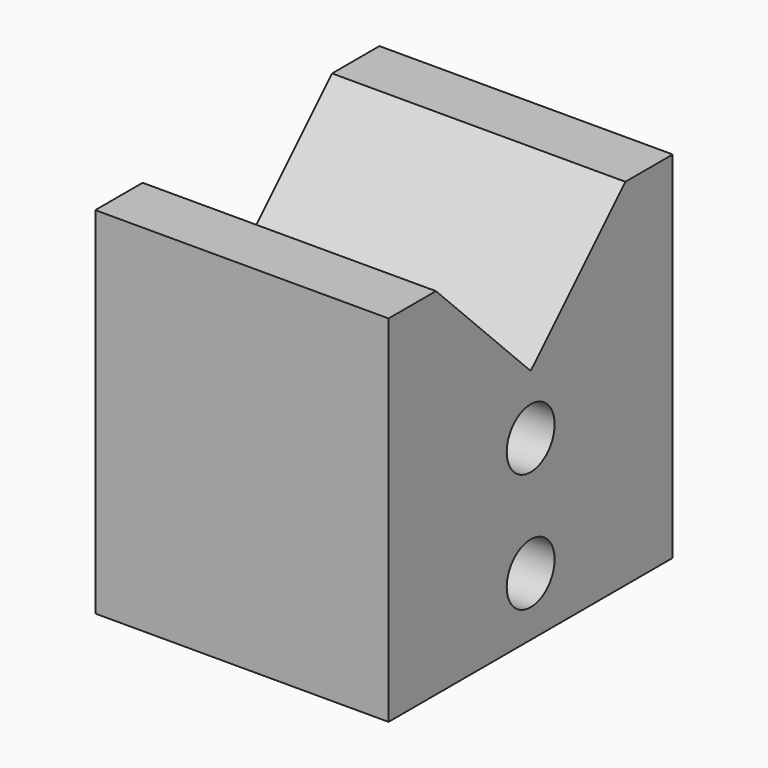
from build123d import *

# Parameters (mm, degrees)
F1_DEPTH = 25
F2_D     = 5.1


# Not quite as in the source:
# - a feature names something its author has since deleted; it is built from what else it names


with BuildPart() as f1:
    # F0 (on Right) → F1 (new body)
    with BuildSketch(Plane.YZ):
        Polygon((24.1157077886, 30.274353966), (19.0699821276, 30.274353966), (19.0699821276, 0), (49.3443360936, 0), (49.3443360936, 30.274353966), (44.2986104326, 30.274353966), (34.2071591106, 20.182902644), align=None)
    extrude(amount=F1_DEPTH)

    # F2 (through all)
    with Locations(Plane(origin=(0, 0, 0), x_dir=(0, 1, 0), z_dir=(-1, 0, 0))):
        with Locations((34.2071591106, -5), (34.2071591106, -15.137176983)):
            Hole(F2_D / 2)


solid = f1.part
